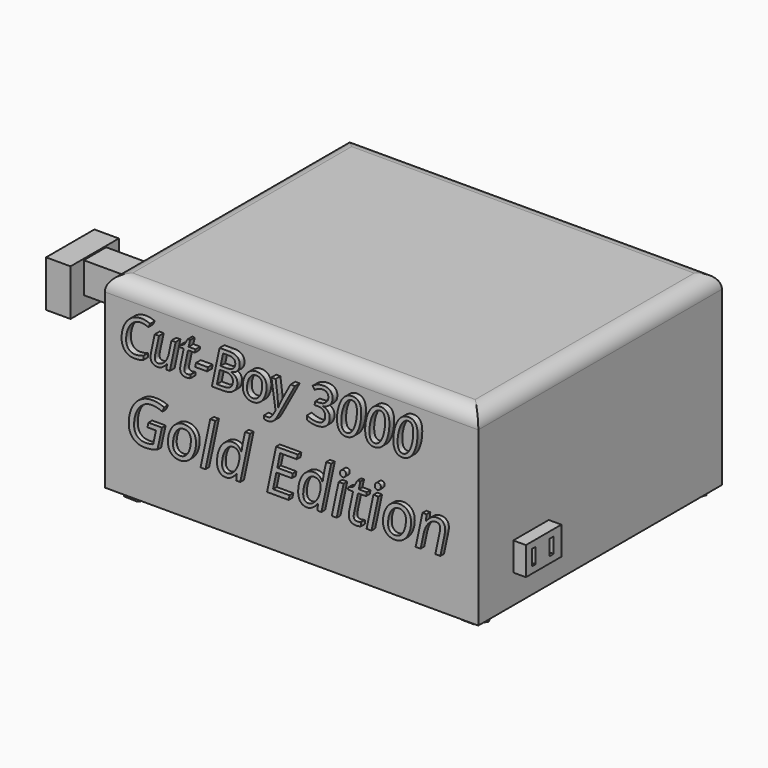
from build123d import *

# Parameters (mm, degrees)
F0_W          = 122.9583881795
F0_H          = 100.2722382545
F1_DEPTH      = 61.81009
F2_R          = 5.08
F5_W          = 52.2091165185
F5_H          = 8.2631036639
F6_DEPTH      = 2.74309
F7_R          = 6.1454081251
F8_DEPTH      = 3.54275
F9_W          = 9.2355473898
F9_H          = 10.1289711893
F10_DEPTH     = 41.92621
F11_W         = 19.8868541047
F11_H         = 15.2589045465
F11_W_2       = 9.2355473898
F11_H_2       = 10.1289711893
F12_DEPTH     = 8.04674
F13_W         = 14.5977977663
F13_H         = 9.3087404966
F14_DEPTH     = 4.1572
F15_W         = 1.4809351414
F15_H         = 5.077493377
F15_W_2       = 1.6924999654
F16_DEPTH     = 25.4
F18_DEPTH     = 1.76366
F20_TEXT_SIZE = 16.8256047699
F21_DEPTH     = 1.95291
F22_TEXT_SIZE = 19.8201767893
F23_DEPTH     = 1.51935


# Not quite as in the source:
# - the program builds the solid bodies; features that only make, move or delete a surface that nothing else refers to are left out
# - Text() gives the source's letters only with a copy of the font that has no kerning and outlines rounded to 1/6400 em; it was checked with that copy


with BuildPart() as f1:
    # F0 (on Top) → F1 (new body)
    with BuildSketch(Plane.XY):
        with Locations((-4.7663990408, 0.9565539658)):
            Rectangle(F0_W, F0_H)
    extrude(amount=F1_DEPTH)

    # F2
    f2_edges = [f1.edges().sort_by_distance(p)[0] for p in [
        (-4.766399, -49.179565, 61.81009),
        (-66.245593, 0.956554, 61.81009),
        (56.712795, 0.956554, 61.81009),
        (-4.766399, 51.092673, 61.81009),
    ]]
    fillet(f2_edges, radius=F2_R)

    # F5 (on face) → F6 (join)
    with BuildSketch(Plane(origin=(0, 51.0926730931, 0), x_dir=(-1, 0, 0), z_dir=(0, 1, 0))):
        with Locations((-11.1125968397, 36.43232584)):
            Rectangle(F5_W, F5_H)
    extrude(amount=F6_DEPTH)

    # F7 (on face) → F8 (join)
    with BuildSketch(Plane(origin=(0, 51.0926730931, 0), x_dir=(-1, 0, 0), z_dir=(0, 1, 0))):
        with Locations((36.4955655017, 37.0090108899)):
            Circle(F7_R)
    extrude(amount=F8_DEPTH)

    # F9 (on face) → F10 (join)
    with BuildSketch(Plane(origin=(-66.2455931306, 0, 0), x_dir=(0, -1, 0), z_dir=(-1, 0, 0))):
        with Locations((0.8481631521, 29.4506344944)):
            Rectangle(F9_W, F9_H)
    extrude(amount=F10_DEPTH)

    # F13 (on face) → F14 (join)
    with BuildSketch(Plane.YZ.offset(56.712795049)):
        with Locations((-27.4863867089, 14.1744762659)):
            Rectangle(F13_W, F13_H)
    extrude(amount=F14_DEPTH)

    # F15 (on face) → F16 (cut)
    with BuildSketch(Plane.YZ.offset(60.869995049)):
        with Locations((-31.5060699359, 14.1744758002)):
            Rectangle(F15_W, F15_H)
        with Locations((-24.2071729153, 14.1744758002)):
            Rectangle(F15_W_2, F15_H)
    extrude(amount=-F16_DEPTH, mode=Mode.SUBTRACT)

    # F17 (on face) → F18 (join)
    with BuildSketch(Plane(origin=(0, 0, 0), x_dir=(1, 0, 0), z_dir=(0, 0, -1))):
        Polygon((53.40458536, -42.3473775793), (48.6322417855, -42.569078505), (47.3683566281, -47.1763563133), (51.3595762174, -49.8021096686), (55.0901707376, -46.8176366801), align=None)
        Polygon((53.2278834429, 46.7441091501), (49.0553639829, 46.7102043331), (46.9984666858, 43.0797440744), (49.1140888486, 39.4831886328), (53.2866083086, 39.5170934498), (55.3435056057, 43.1475537085), align=None)
        Polygon((-56.5425550613, 39.4001904598), (-54.3985888362, 43.5367748141), (-56.9089928594, 47.4617962071), (-61.5633631077, 47.2502332458), (-63.7073293328, 43.1136488914), (-61.1969253096, 39.1886274985), align=None)
        Polygon((-56.5294037624, -48.8855687799), (-56.302651763, -45.1078228652), (-59.4608996944, -43.022576916), (-62.8458996252, -44.7150768815), (-63.0726516247, -48.4928227961), (-59.9144036933, -50.5780687453), align=None)
    extrude(amount=F18_DEPTH)

    # F20 (on face) → F21 (join)
    with BuildSketch(Plane.XZ.offset(49.1795651615)):
        with Locations((-60.4162588716, 42.0819632709)):
            Text('Cut-Boy 3000', F20_TEXT_SIZE, font='Open Sans', font_style=FontStyle.ITALIC, text_align=(TextAlign.LEFT, TextAlign.BOTTOM))
    extrude(amount=F21_DEPTH)

    # F22 (on face) → F23 (join)
    with BuildSketch(Plane.XZ.offset(49.1795651615)):
        with Locations((-58.6210377514, 17.1088185161)):
            Text('Gold Edition', F22_TEXT_SIZE, font='Open Sans', font_style=FontStyle.ITALIC, text_align=(TextAlign.LEFT, TextAlign.BOTTOM))
    extrude(amount=F23_DEPTH)


with BuildPart() as f12:
    # F11 (on face) → F12 (new body)
    with BuildSketch(Plane(origin=(-108.1718031306, 0, 0), x_dir=(0, -1, 0), z_dir=(-1, 0, 0))):
        with Locations((0.9687379934, 27.3228976876)):
            Rectangle(F11_W, F11_H)
        with Locations((0.8481631521, 29.4506344944)):
            Rectangle(F11_W_2, F11_H_2, mode=Mode.SUBTRACT)
    extrude(amount=F12_DEPTH)


solid = Compound([f1.part, f12.part])
